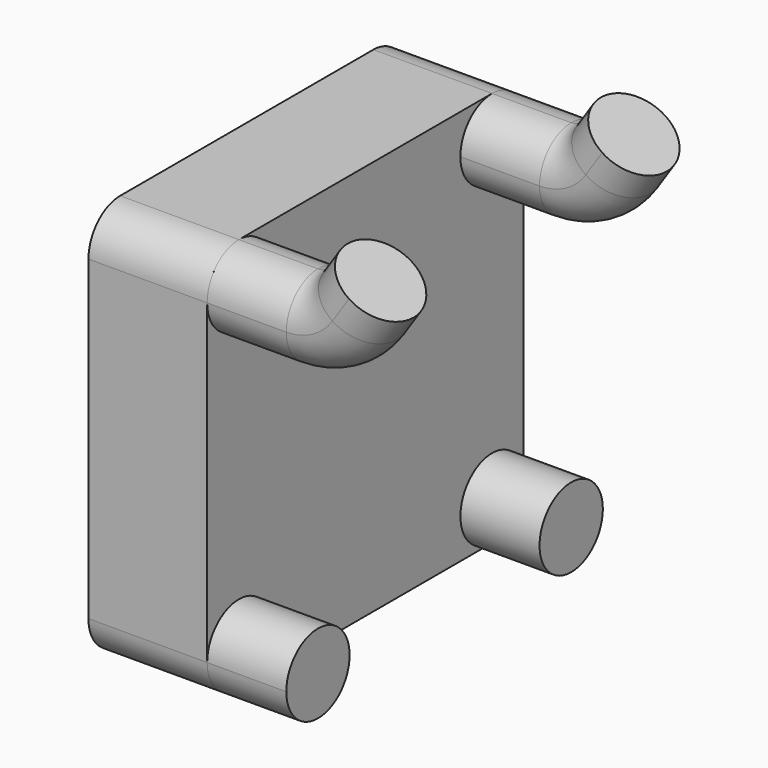
from build123d import *

# Parameters (mm, degrees)
F0_W      = 31.75
F0_H      = 31.75
F1_DEPTH  = 9.525
F10_DEPTH = 6.35
F11_R     = 3.1749


# Not quite as in the source:
# - a fillet or chamfer is up to 0.001 mm smaller than in the source, because OpenCascade refuses the exact size


with BuildPart() as f1:
    # F0 (on Right) → F1 (new body)
    with BuildSketch(Plane.YZ):
        Rectangle(F0_W, F0_H)
    extrude(amount=F1_DEPTH)

    # F6: sweep along a path in F5
    with BuildLine(Plane.XZ.offset(12.7)) as f6_path:
        Line((9.525, 9.525), (15.875, 9.525))
        ThreePointArc((15.875, 9.525), (19.4783384003, 10.4308096264), (22.225, 12.9328865162))
        Line((22.225, 12.9328865162), (23.5505334947, 14.9312034475))
    # F2 (on face) → F6 (sweep)
    with BuildSketch(Plane.YZ.offset(9.525)):
        with BuildLine():
            ThreePointArc((-15.875, 12.7), (-12.7, 9.525), (-9.525, 12.7))
            ThreePointArc((-9.525, 12.7), (-10.4549359718, 14.9450640323), (-12.7000000057, 15.875))
            ThreePointArc((-12.7000000057, 15.875), (-14.9450640323, 14.9450640282), (-15.875, 12.7))
        make_face()
    sweep(path=f6_path.line)

    # F9: F1 across plane


with BuildPart() as f1_1:
    add(f1.part)
    add(f1.part.mirror(Plane(origin=(0, 0, 15.875), x_dir=(1, 0, 0), z_dir=(0, -1, 0))))

    # F2 (on face) → F10 (join)
    with BuildSketch(Plane.YZ.offset(9.525)):
        with BuildLine():
            ThreePointArc((-9.525, -12.7), (-12.7, -9.525), (-15.875, -12.7))
            ThreePointArc((-15.875, -12.7), (-14.9450640303, -14.9450640303), (-12.7, -15.875))
            ThreePointArc((-12.7, -15.875), (-10.4549359697, -14.9450640303), (-9.525, -12.7))
        make_face()
        with BuildLine():
            ThreePointArc((12.7, -15.875), (14.9450640303, -14.9450640303), (15.875, -12.7))
            ThreePointArc((15.875, -12.7), (10.4549359697, -10.4549359697), (12.7, -15.875))
        make_face()
    extrude(amount=F10_DEPTH)

    # F11 (radius 3.175 in the source; OpenCascade refuses exactly that, so slightly less here)
    f11_edges = [f1_1.edges().sort_by_distance(p)[0] for p in [
        (4.7625, -15.875, 15.875),
        (4.7625, -15.875, -15.875),
        (4.7625, 15.875, -15.875),
        (4.7625, 15.875, 15.875),
    ]]
    fillet(f11_edges, radius=F11_R)


solid = f1_1.part
